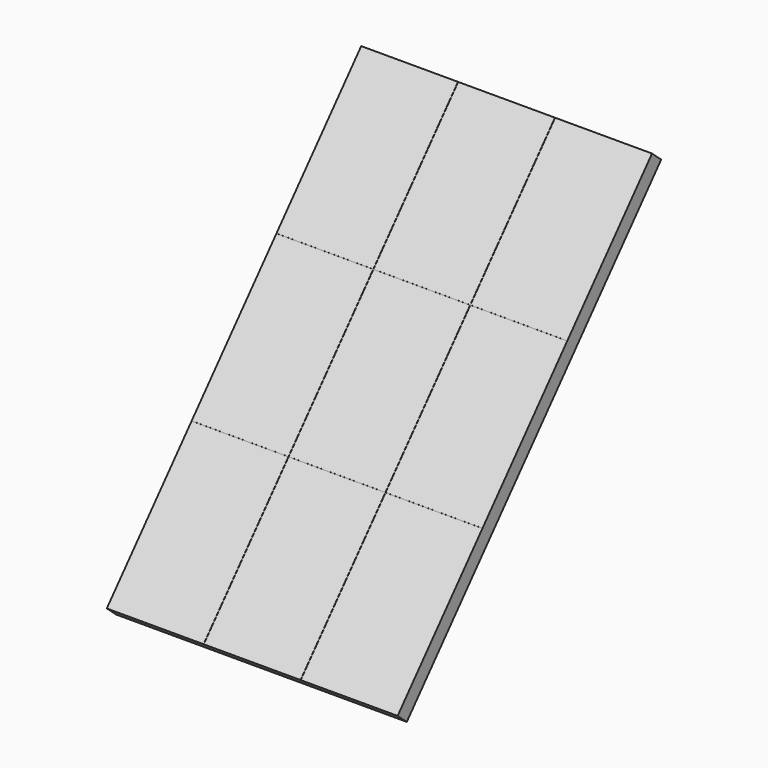
from build123d import *

# Parameters (mm, degrees)
F1_DEPTH = 2948.94
F2_W     = 981.71
F2_H     = 1.27
F2_W_2   = 1.27
F2_H_2   = 1637.03
F2_H_3   = 1635.76
F2_W_3   = 980.44
F3_DEPTH = 2.54
F4_DEPTH = 2.54


with BuildPart() as f1:
    # F0 (on Right) → F1 (new body)
    with BuildSketch(Plane.YZ):
        Polygon((-2936.1038094659, -2649.6760176359), (0, 727.9250450949), (288.3607121196, 1059.646098201), (172.00109846, 1160.7959671727), (-3052.4634231254, -2548.5261486642), align=None)
    extrude(amount=F1_DEPTH)

    # F2 (on face) → F3 (cut)
    with BuildSketch(Plane(origin=(0, -476.780077957, 414.458598623), x_dir=(1, 0, 0), z_dir=(0, -0.7547095802, 0.656059029))):
        with Locations((490.855, -648.7582892498)):
            Rectangle(F2_W, F2_H)
        with Locations((982.345, 170.3917107502)):
            Rectangle(F2_W_2, F2_H_2)
        with Locations((490.855, -650.0282892498)):
            Rectangle(F2_W, F2_H)
        with Locations((982.345, -648.7582892498)):
            Rectangle(F2_W_2, F2_H)
        with Locations((983.615, 170.3917107502)):
            Rectangle(F2_W_2, F2_H_2)
        with Locations((982.345, -650.0282892498)):
            Rectangle(F2_W_2, F2_H)
        with Locations((983.615, -648.7582892498)):
            Rectangle(F2_W_2, F2_H)
        with Locations((490.855, -2287.0582892498)):
            Rectangle(F2_W, F2_H)
        with Locations((982.345, -1468.5432892498)):
            Rectangle(F2_W_2, F2_H_3)
        with Locations((983.615, -650.0282892498)):
            Rectangle(F2_W_2, F2_H)
        with Locations((1474.47, -648.7582892498)):
            Rectangle(F2_W_3, F2_H)
        with Locations((1965.325, 170.3917107502)):
            Rectangle(F2_W_2, F2_H_2)
        with Locations((982.345, -2287.0582892498)):
            Rectangle(F2_W_2, F2_H)
        with Locations((983.615, -1468.5432892498)):
            Rectangle(F2_W_2, F2_H_3)
        with Locations((1474.47, -650.0282892498)):
            Rectangle(F2_W_3, F2_H)
        with Locations((1965.325, -648.7582892498)):
            Rectangle(F2_W_2, F2_H)
        with Locations((1966.595, 170.3917107502)):
            Rectangle(F2_W_2, F2_H_2)
        with Locations((982.345, -2288.3282892498)):
            Rectangle(F2_W_2, F2_H)
        with Locations((983.615, -2287.0582892498)):
            Rectangle(F2_W_2, F2_H)
        with Locations((1965.325, -650.0282892498)):
            Rectangle(F2_W_2, F2_H)
        with Locations((1966.595, -648.7582892498)):
            Rectangle(F2_W_2, F2_H)
        with Locations((983.615, -2288.3282892498)):
            Rectangle(F2_W_2, F2_H)
        with Locations((1966.595, -650.0282892498)):
            Rectangle(F2_W_2, F2_H)
    extrude(amount=-F3_DEPTH, mode=Mode.SUBTRACT)

    # F2 (on face) → F4 (cut)
    with BuildSketch(Plane(origin=(0, -476.780077957, 414.458598623), x_dir=(1, 0, 0), z_dir=(0, -0.7547095802, 0.656059029))):
        with Locations((490.855, -2288.3282892498)):
            Rectangle(F2_W, F2_H)
        with Locations((983.615, -3107.4782892498)):
            Rectangle(F2_W_2, F2_H_2)
        with Locations((982.345, -3107.4782892498)):
            Rectangle(F2_W_2, F2_H_2)
        with Locations((982.345, -2288.3282892498)):
            Rectangle(F2_W_2, F2_H)
        with Locations((1474.47, -2288.3282892498)):
            Rectangle(F2_W_3, F2_H)
        with Locations((1474.47, -2287.0582892498)):
            Rectangle(F2_W_3, F2_H)
        with Locations((2458.085, -648.7582892498)):
            Rectangle(F2_W, F2_H)
        with Locations((2458.085, -650.0282892498)):
            Rectangle(F2_W, F2_H)
        with Locations((1966.595, -1468.5432892498)):
            Rectangle(F2_W_2, F2_H_3)
        with Locations((1965.325, -1468.5432892498)):
            Rectangle(F2_W_2, F2_H_3)
        with Locations((1965.325, -2287.0582892498)):
            Rectangle(F2_W_2, F2_H)
        with Locations((1965.325, -2288.3282892498)):
            Rectangle(F2_W_2, F2_H)
        with Locations((1966.595, -2287.0582892498)):
            Rectangle(F2_W_2, F2_H)
        with Locations((1966.595, -2288.3282892498)):
            Rectangle(F2_W_2, F2_H)
        with Locations((2458.085, -2287.0582892498)):
            Rectangle(F2_W, F2_H)
        with Locations((1965.325, -3107.4782892498)):
            Rectangle(F2_W_2, F2_H_2)
        with Locations((1966.595, -3107.4782892498)):
            Rectangle(F2_W_2, F2_H_2)
        with Locations((2458.085, -2288.3282892498)):
            Rectangle(F2_W, F2_H)
    extrude(amount=-F4_DEPTH, mode=Mode.SUBTRACT)


solid = f1.part
